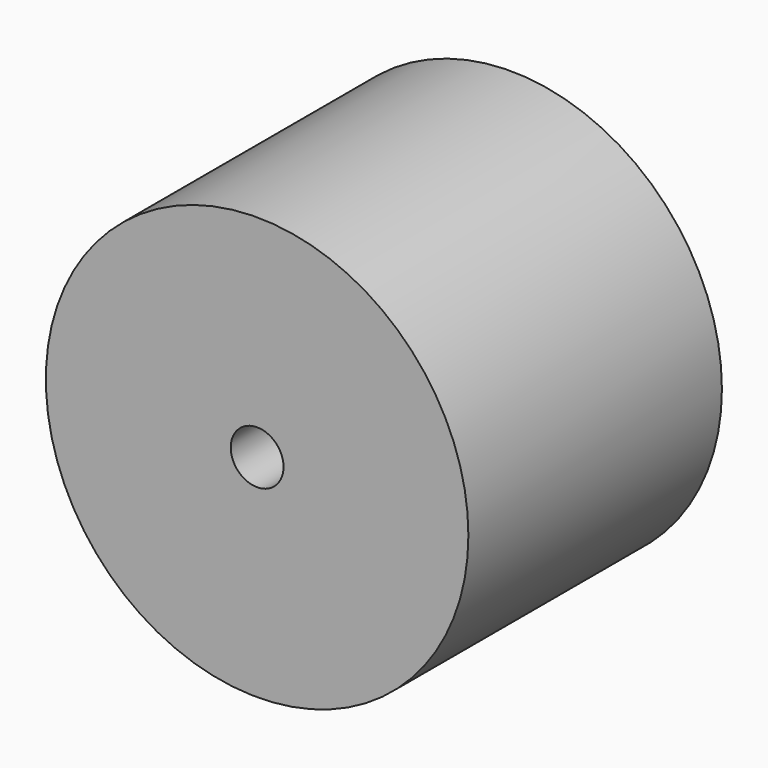
from build123d import *

# Parameters (mm, degrees)
F0_R     = 25.4
F0_R_2   = 3.175
F1_DEPTH = 38.1


# Not quite as in the source:
# - the program builds the solid bodies; features that only make, move or delete a surface that nothing else refers to are left out


with BuildPart() as f1:
    # F0 (on Front) → F1 (new body)
    with BuildSketch(Plane.XZ):
        Circle(F0_R)
        Circle(F0_R_2, mode=Mode.SUBTRACT)
    extrude(amount=F1_DEPTH)


solid = f1.part
